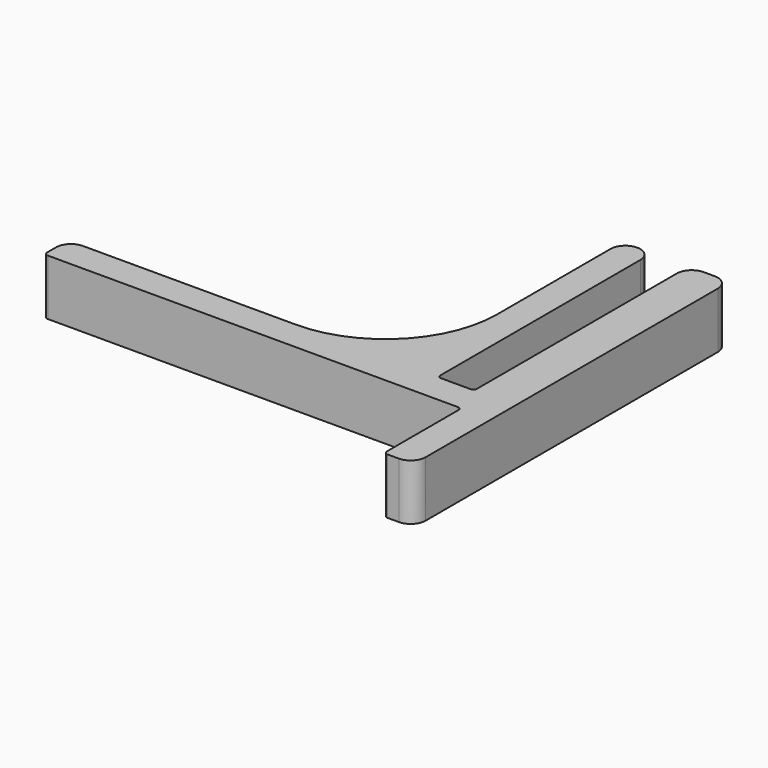
from build123d import *

# Parameters (mm, degrees)
F1_DEPTH = 7.5
F2_R     = 1.99999
F3_R     = 15
F4_R     = 0.5


# Not quite as in the source:
# - a fillet or chamfer is up to 0.001 mm smaller than in the source, because OpenCascade refuses the exact size


with BuildPart() as f1:
    # F0 (on Top) → F1 (new body)
    with BuildSketch(Plane.XY):
        Polygon((45.6, 4), (0, 4), (0, 0), (56, 0), (56, -13), (60, -13), (60, 40), (54.5, 40), (54.5, 4), (49.6, 4), (49.6, 40), (45.6, 40), align=None)
    extrude(amount=F1_DEPTH)

    # F2 (radius 2 in the source; OpenCascade refuses exactly that, so slightly less here)
    f2_edges = [f1.edges().sort_by_distance(p)[0] for p in [
        (60, -13, 3.75),
        (60, 40, 3.75),
        (54.5, 40, 3.75),
        (49.6, 40, 3.75),
        (45.6, 40, 3.75),
        (0, 4, 3.75),
    ]]
    fillet(f2_edges, radius=F2_R)

    # F3
    f3_edges = [f1.edges().sort_by_distance(p)[0] for p in [
        (45.6, 4, 3.75),
    ]]
    fillet(f3_edges, radius=F3_R)

    # F4
    f4_edges = [f1.edges().sort_by_distance(p)[0] for p in [
        (49.6, 4, 3.75),
        (54.5, 4, 3.75),
        (0, 0, 3.75),
        (56, -13, 3.75),
        (56, 0, 3.75),
    ]]
    fillet(f4_edges, radius=F4_R)


solid = f1.part
